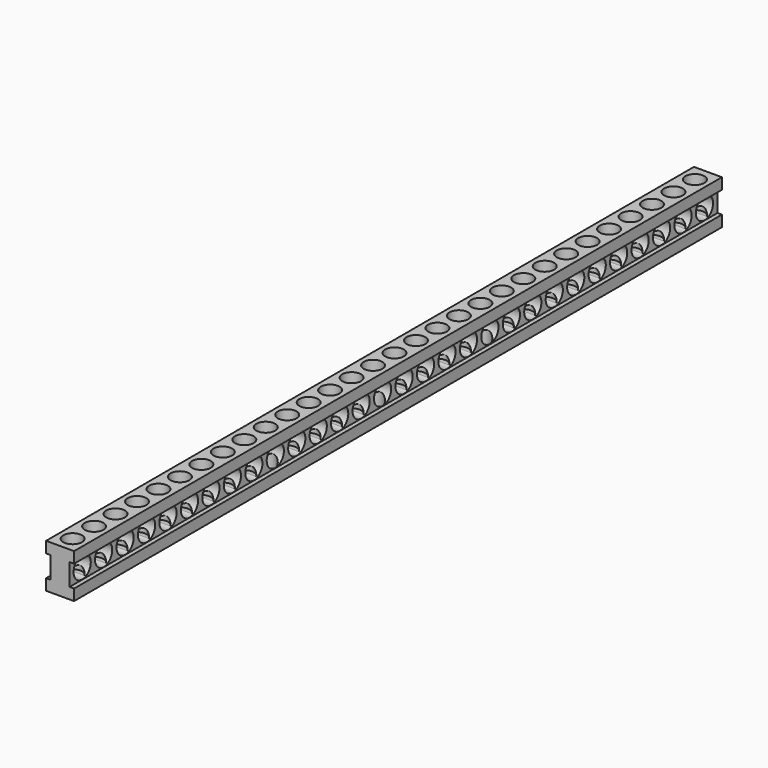
from build123d import *

# Parameters (mm, degrees)
F1_DEPTH = 237.3
F2_R     = 3.15
F3_DEPTH = 6.901
F4_R     = 2.75
F5_DEPTH = 9.3
F6_DEPTH = 12.901


# Not quite as in the source:
# - a feature names something its author has since deleted; it is built from what else it names


with BuildPart() as f1:
    # F0 (on Front) → F1 (new body)
    with BuildSketch(Plane.XZ):
        Polygon((0, 3.25), (0, 0), (8.2, 0), (8.2, 3.25), (6.9, 3.25), (6.9, 9.65), (8.2, 9.65), (8.2, 12.9), (0, 12.9), (0, 9.65), (1.3, 9.65), (1.3, 3.25), align=None)
    extrude(amount=F1_DEPTH)

    # F2 (on face) → F3 (cut, through all)
    with BuildSketch(Plane.YZ.offset(6.9)):
        with Locations((-232.7, 6.45)):
            Circle(F2_R)
        with Locations((-224.84, 6.45)):
            Circle(F2_R)
        with Locations((-216.98, 6.45)):
            Circle(F2_R)
        with Locations((-209.12, 6.45)):
            Circle(F2_R)
        with Locations((-201.26, 6.45)):
            Circle(F2_R)
        with Locations((-193.4, 6.45)):
            Circle(F2_R)
        with Locations((-185.54, 6.45)):
            Circle(F2_R)
        with Locations((-177.68, 6.45)):
            Circle(F2_R)
        with Locations((-169.82, 6.45)):
            Circle(F2_R)
        with Locations((-161.96, 6.45)):
            Circle(F2_R)
        with Locations((-154.1, 6.45)):
            Circle(F2_R)
        with Locations((-146.24, 6.45)):
            Circle(F2_R)
        with Locations((-138.38, 6.45)):
            Circle(F2_R)
        with Locations((-130.52, 6.45)):
            Circle(F2_R)
        with Locations((-122.66, 6.45)):
            Circle(F2_R)
        with Locations((-114.8, 6.45)):
            Circle(F2_R)
        with Locations((-106.94, 6.45)):
            Circle(F2_R)
        with Locations((-99.08, 6.45)):
            Circle(F2_R)
        with Locations((-91.22, 6.45)):
            Circle(F2_R)
        with Locations((-83.36, 6.45)):
            Circle(F2_R)
        with Locations((-75.5, 6.45)):
            Circle(F2_R)
        with Locations((-67.64, 6.45)):
            Circle(F2_R)
        with Locations((-59.78, 6.45)):
            Circle(F2_R)
        with Locations((-51.92, 6.45)):
            Circle(F2_R)
        with Locations((-44.06, 6.45)):
            Circle(F2_R)
        with Locations((-36.2, 6.45)):
            Circle(F2_R)
        with Locations((-28.34, 6.45)):
            Circle(F2_R)
        with Locations((-20.48, 6.45)):
            Circle(F2_R)
        with Locations((-12.62, 6.45)):
            Circle(F2_R)
        with Locations((-4.76, 6.45)):
            Circle(F2_R)
    extrude(amount=-F3_DEPTH, mode=Mode.SUBTRACT)

    # F4 (on face) → F5 (cut)
    with BuildSketch(Plane.XY.offset(12.9)):
        with Locations((4.1, -232.7)):
            Circle(F4_R)
        with Locations((4.1, -224.84)):
            Circle(F4_R)
        with Locations((4.1, -216.98)):
            Circle(F4_R)
        with Locations((4.1, -209.12)):
            Circle(F4_R)
        with Locations((4.1, -201.26)):
            Circle(F4_R)
        with Locations((4.1, -193.4)):
            Circle(F4_R)
        with Locations((4.1, -185.54)):
            Circle(F4_R)
        with Locations((4.1, -177.68)):
            Circle(F4_R)
        with Locations((4.1, -169.82)):
            Circle(F4_R)
        with Locations((4.1, -154.1)):
            Circle(F4_R)
        with Locations((4.1, -146.24)):
            Circle(F4_R)
        with Locations((4.1, -138.38)):
            Circle(F4_R)
        with Locations((4.1, -130.52)):
            Circle(F4_R)
        with Locations((4.1, -114.8)):
            Circle(F4_R)
        with Locations((4.1, -106.94)):
            Circle(F4_R)
        with Locations((4.1, -99.08)):
            Circle(F4_R)
        with Locations((4.1, -91.22)):
            Circle(F4_R)
        with Locations((4.1, -75.5)):
            Circle(F4_R)
        with Locations((4.1, -67.64)):
            Circle(F4_R)
        with Locations((4.1, -59.78)):
            Circle(F4_R)
        with Locations((4.1, -51.92)):
            Circle(F4_R)
        with Locations((4.1, -44.06)):
            Circle(F4_R)
        with Locations((4.1, -36.2)):
            Circle(F4_R)
        with Locations((4.1, -28.34)):
            Circle(F4_R)
        with Locations((4.1, -20.48)):
            Circle(F4_R)
        with Locations((4.1, -12.62)):
            Circle(F4_R)
        with Locations((4.1, -4.76)):
            Circle(F4_R)
    extrude(amount=-F5_DEPTH, mode=Mode.SUBTRACT)

    # F4 (on face) → F6 (cut, through all)
    with BuildSketch(Plane.XY.offset(12.9)):
        with Locations((4.1, -161.96)):
            Circle(F4_R)
        with Locations((4.1, -122.66)):
            Circle(F4_R)
        with Locations((4.1, -83.36)):
            Circle(F4_R)
    extrude(amount=-F6_DEPTH, mode=Mode.SUBTRACT)


solid = f1.part
